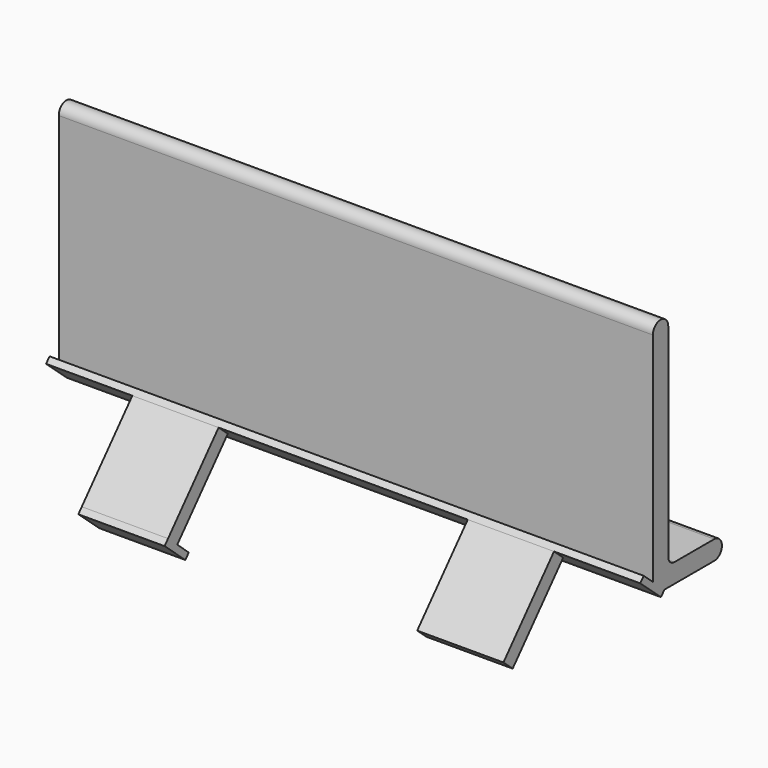
from build123d import *

# Parameters (mm, degrees)
F1_DEPTH = 155
F3_DEPTH = 155
F5_START = 22.5
F5_DEPTH = 22.5
F6_START = 110
F6_DEPTH = 22.5
F8_START = 22.5
F8_DEPTH = 22.5


# Not quite as in the source:
# - a feature of the source that left no trace in its solid (it failed there, or was rolled back) is left out


with BuildPart() as f1:
    # F0 (on Right) → F1 (new body)
    with BuildSketch(Plane.YZ):
        with BuildLine():
            Line((-25.3971134126, 39.5229434967), (-30.3971134126, 39.5229434967))
            Line((-30.3971134126, 39.5229434967), (-30.3971134126, -18.4770565033))
            ThreePointArc((-30.3971134126, -18.4770565033), (-29.811326975, -19.8912700657), (-28.3971134126, -20.4770565033))
            Line((-28.3971134126, -20.4770565033), (-10.3971134126, -20.4770565033))
            Line((-10.3971134126, -20.4770565033), (-10.3971134126, -15.4770565033))
            Line((-10.3971134126, -15.4770565033), (-23.3971134126, -15.4770565033))
            ThreePointArc((-23.3971134126, -15.4770565033), (-24.811326975, -14.8912700657), (-25.3971134126, -13.4770565033))
            Line((-25.3971134126, -13.4770565033), (-25.3971134126, 39.5229434967))
        make_face()
        with BuildLine():
            ThreePointArc((-25.3971134126, 39.5229434967), (-27.8971134126, 42.0229434967), (-30.3971134126, 39.5229434967))
            Line((-30.3971134126, 39.5229434967), (-25.3971134126, 39.5229434967))
        make_face()
        with BuildLine():
            Line((-10.3971134126, -15.4770565033), (-10.3971134126, -20.4770565033))
            ThreePointArc((-10.3971134126, -20.4770565033), (-7.8971134126, -17.9770565033), (-10.3971134126, -15.4770565033))
        make_face()
    extrude(amount=F1_DEPTH)

    # F2 (on Right) → F3 (join)
    with BuildSketch(Plane.YZ):
        Polygon((-26.6438154831, -20.4771793517), (-33.4096477321, -14.5422392527), (-34.530691973, -15.8202297886), (-27.764859724, -21.7551698876), align=None)
    extrude(amount=F3_DEPTH)

    # F4 (on Right) → F5 (join)
    with BuildSketch(Plane.YZ.offset(F5_START)):
        Polygon((-31.5236554179, -18.4579809437), (-34.530691973, -15.8202297886), (-51.0166366924, -34.614208258), (-48.0096001373, -37.2519594131), align=None)
    extrude(amount=F5_DEPTH)

    # F4 (on Right) → F6 (join)
    with BuildSketch(Plane.YZ.offset(F6_START)):
        Polygon((-31.5236554179, -18.4579809437), (-34.530691973, -15.8202297886), (-51.0166366924, -34.614208258), (-48.0096001373, -37.2519594131), align=None)
    extrude(amount=F6_DEPTH)

    # F7 (on Right) → F8 (join)
    with BuildSketch(Plane.YZ.offset(F8_START)):
        Polygon((-51.0166366924, -34.614208258), (-52.136497942, -35.8932355375), (-45.370665693, -41.8281756365), (-44.2508044434, -40.549148357), align=None)
    extrude(amount=F8_DEPTH)


solid = f1.part
